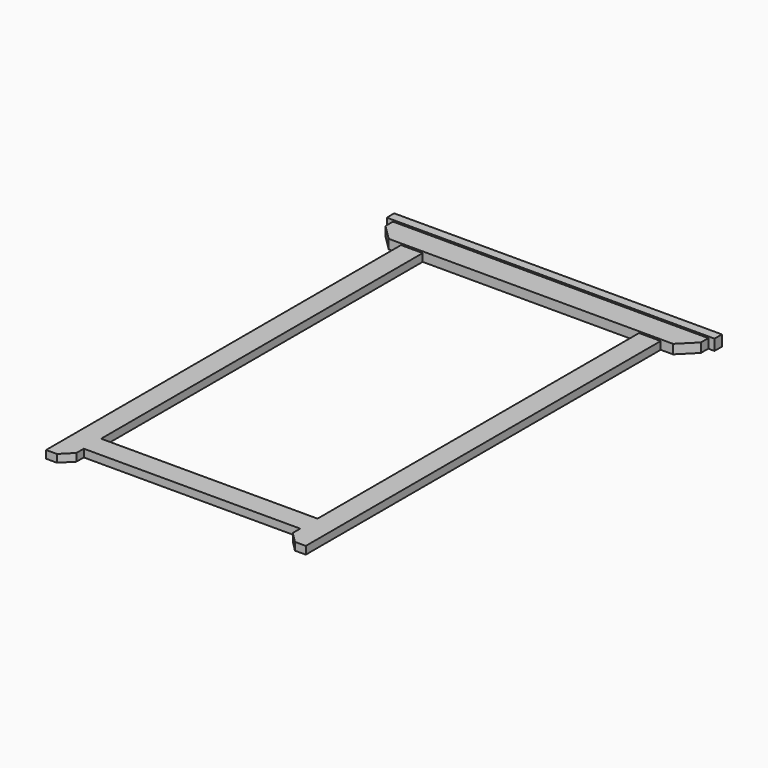
from build123d import *

# Parameters (mm, degrees)
F1_DEPTH = 30
F0_W     = 20
F0_H     = 30
F0_W_2   = 1020
F2_DEPTH = 35
F0_W_3   = 700
F0_H_2   = 70
F3_DEPTH = 25


with BuildPart() as f1:
    # F0 (on Top) → F1 (new body)
    with BuildSketch(Plane.XY):
        Polygon((-1947.5297451019, -160.4416549206), (-1877.5297451019, -160.4416549206), (-1177.5297451019, -160.4416549206), (-1107.5297451019, -160.4416549206), (-1067.5297451019, -160.4416549206), (-1017.5297451019, -110.4416549206), (-1017.5297451019, -80.4416549206), (-2037.5297451019, -80.4416549206), (-2037.5297451019, -110.4416549206), (-1987.5297451019, -160.4416549206), align=None)
    extrude(amount=F1_DEPTH)

    # F0 (on Top) → F2 (join)
    with BuildSketch(Plane.XY):
        with Locations((-2047.5297451019, -65.4416549206)):
            Rectangle(F0_W, F0_H)
        with Locations((-1527.5297451019, -65.4416549206)):
            Rectangle(F0_W_2, F0_H)
        with Locations((-1007.5297451019, -65.4416549206)):
            Rectangle(F0_W, F0_H)
    extrude(amount=F2_DEPTH)

    # F0 (on Top) → F3 (join)
    with BuildSketch(Plane.XY):
        Polygon((-1877.5297451019, -1460.4416549206), (-1877.5297451019, -160.4416549206), (-1947.5297451019, -160.4416549206), (-1947.5297451019, -1595.4416549206), (-1912.5297451019, -1595.4416549206), (-1877.5297451019, -1560.4416549206), (-1877.5297451019, -1530.4416549206), align=None)
        with Locations((-1527.5297451019, -1495.4416549206)):
            Rectangle(F0_W_3, F0_H_2)
        Polygon((-1107.5297451019, -160.4416549206), (-1177.5297451019, -160.4416549206), (-1177.5297451019, -1460.4416549206), (-1177.5297451019, -1530.4416549206), (-1177.5297451019, -1560.4416549206), (-1142.5297451019, -1595.4416549206), (-1107.5297451019, -1595.4416549206), align=None)
    extrude(amount=F3_DEPTH)


solid = f1.part
